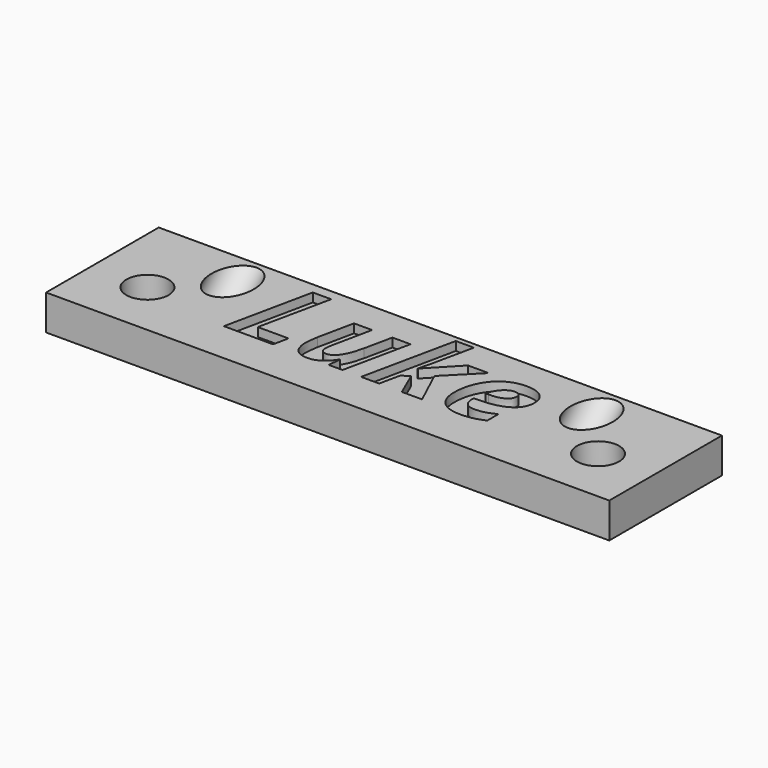
from build123d import *

# Parameters (mm, degrees)
F0_W         = 101.6
F0_H         = 25.4
F1_DEPTH     = 6.35
F2_R         = 3.81
F3_DEPTH     = 25.4
F7_R         = 3.81
F8_DEPTH     = 62.8627928475
F9_TEXT_SIZE = 22.212201954
F10_DEPTH    = 1.5875


# Not quite as in the source:
# - Text() gives the source's letters only with a copy of the font that has no kerning and outlines rounded to 1/6400 em; it was checked with that copy


with BuildPart() as f1:
    # F0 (on Top) → F1 (new body)
    with BuildSketch(Plane.XY):
        Rectangle(F0_W, F0_H)
    extrude(amount=F1_DEPTH)

    # F2 (on face) → F3 (cut)
    with BuildSketch(Plane.XY.offset(6.35)):
        with Locations((-40.64, -2.54)):
            Circle(F2_R)
        with Locations((40.64, -2.54)):
            Circle(F2_R)
    extrude(amount=-F3_DEPTH, mode=Mode.SUBTRACT)

    # F7 (on 3pt) → F8 (cut, through all)
    with BuildSketch(Plane(origin=(0, 38.1, 38.1), x_dir=(1, 0, 0), z_dir=(0, -0.7071067812, -0.7071067812))):
        with Locations((-32.385, 0)):
            Circle(F7_R)
        with Locations((32.385, 0)):
            Circle(F7_R)
    extrude(amount=F8_DEPTH, mode=Mode.SUBTRACT)

    # F9 (on face) → F10 (cut)
    with BuildSketch(Plane.XY.offset(6.35)):
        with Locations((-25.4, -5.08)):
            Text('Luke', F9_TEXT_SIZE, font='Open Sans', font_style=FontStyle.BOLDITALIC, text_align=(TextAlign.LEFT, TextAlign.BOTTOM))
    extrude(amount=-F10_DEPTH, mode=Mode.SUBTRACT)


solid = f1.part
